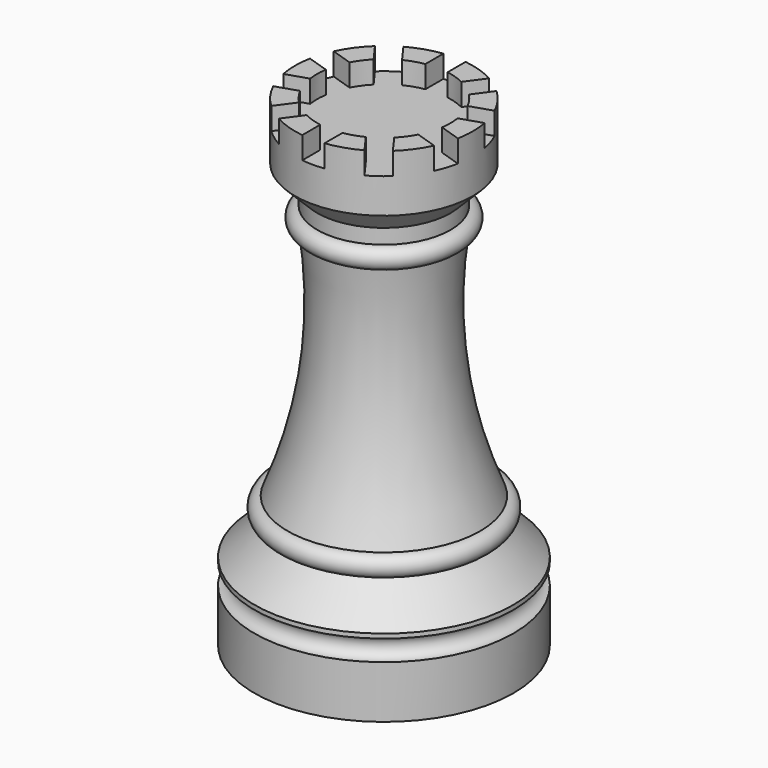
from build123d import *

# Parameters (mm, degrees)
F4_W            = 3.81
F4_H            = 3.81
F5_DEPTH        = 22.226
F5_DEPTH_BACK   = 22.226
F5_COPIES_COUNT = 5
F5_COPIES_ANGLE = 144


# Not quite as in the source:
# - a feature of the source that left no trace in its solid (it failed there, or was rolled back) is left out
# - a pattern or mirror of a feature is missing from the dataset's text; its kind, count and spacing are read off the source's solid


with BuildPart() as f1:
    # F0 (on Front) → F1 (revolve)
    with BuildSketch(Plane.XZ):
        with BuildLine():
            Line((16.51, 0), (0, 0))
            Line((0, 0), (0, -19.05))
            Line((0, -19.05), (22.225, -19.05))
            Line((22.225, -19.05), (22.225, -10.033))
            ThreePointArc((22.225, -10.033), (20.447, -8.255), (22.225, -6.477))
            Line((22.225, -6.477), (22.225, -5.715))
            Line((22.225, -5.715), (16.51, 0))
        make_face()
    revolve(axis=Axis((0, 0, -9.525), (0, 0, 1)))

    # F2 (on Front) → F3 (revolve)
    with BuildSketch(Plane.XZ):
        with BuildLine():
            Line((0, 59.69), (0, 0))
            Line((0, 0), (16.51, 0))
            ThreePointArc((16.51, 0), (18.288, 1.778), (16.51, 3.556))
            ThreePointArc((16.51, 3.556), (11.2408861288, 23.3411323191), (11.43, 43.815))
            ThreePointArc((11.43, 43.815), (13.208, 45.593), (11.43, 47.371))
            Line((11.43, 47.371), (11.43, 49.911))
            Line((11.43, 49.911), (15.24, 53.721))
            Line((15.24, 53.721), (15.24, 63.5))
            Line((15.24, 63.5), (11.43, 63.5))
            Line((11.43, 63.5), (11.43, 59.69))
            Line((11.43, 59.69), (0, 59.69))
        make_face()
    revolve(axis=Axis((0, 0, 29.845), (0, 0, 1)))

    # F4 (on Front) → F5 (cut, two sides)
    with BuildSketch(Plane.XZ) as f5_sk:
        with Locations((0, 61.595)):
            Rectangle(F4_W, F4_H)
    f5 = extrude(amount=F5_DEPTH, mode=Mode.SUBTRACT) + extrude(f5_sk.sketch, amount=-F5_DEPTH_BACK, mode=Mode.SUBTRACT)

    # F5_copies: F5 ×5 about axis
    f5_copies_axis = Axis((0, 0, 0), (0, 0, 1))
    for i in range(1, F5_COPIES_COUNT):
        add(f5.rotate(f5_copies_axis, i * F5_COPIES_ANGLE / (F5_COPIES_COUNT - 1)), mode=Mode.SUBTRACT)


solid = f1.part
